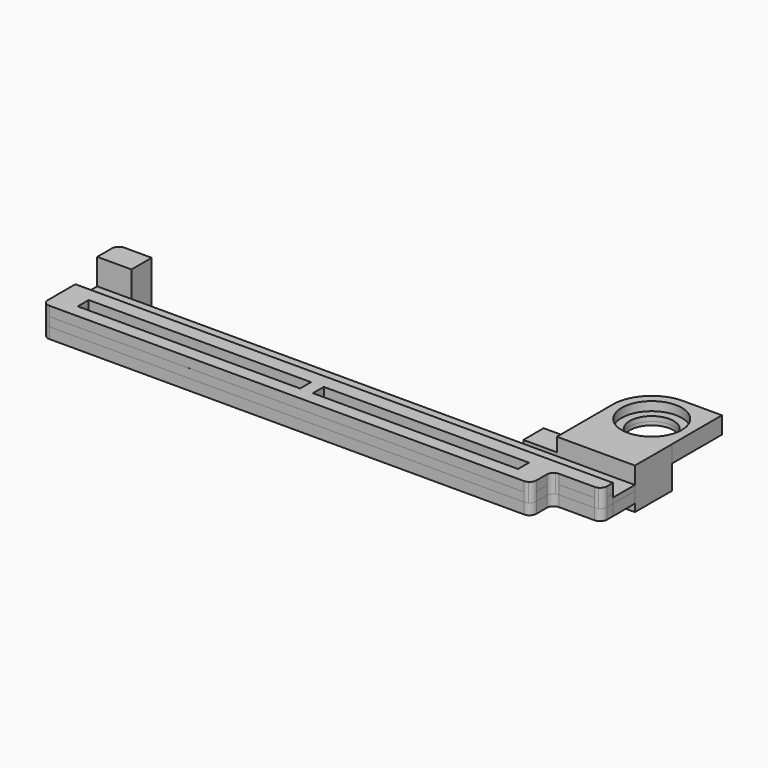
from build123d import *

# Parameters (mm, degrees)
F0_W           = 32.5
F0_H           = 2
F0_W_2         = 30
F1_DEPTH       = 1.4
F3_DEPTH       = 1.3
F4_DEPTH       = 1.6
F5_W           = 67
F5_H           = 6.7
F6_DEPTH       = 4.301
F9_T4_DEPTH    = 3.9
F9_T9_DEPTH    = 3.8
F9_T11_DEPTH   = 6.3
F9_T13_DEPTH   = 6.4
F9_2_F1_R      = 1
F9_2_F2_R      = 1
F11_DEPTH      = 4
F12_R          = 4.4
F13_DEPTH      = 2
F12_R_2        = 3.2
F14_DEPTH      = 0.7
F15_DEPTH      = 0.5
F7_W           = 5
F7_H           = 3.7
F16_DEPTH      = 3.3
F16_DEPTH_BACK = 2.9
F8_W           = 4.9
F8_H           = 3.7
F17_DEPTH      = 6
F19_DEPTH      = 0.5
F20_R          = 1


# Not quite as in the source:
# - a fillet or chamfer that OpenCascade refuses, or shapes differently, is made with other operations: its cross-section is extruded or revolved along the edge and cut away or added
# - ends of sketch curves that miss each other by under 0.0002 mm in the source are joined


with BuildPart() as f1:
    # F0 (on Top) → F1 (new body)
    with BuildSketch(Plane.XY):
        Polygon((78.6000193149, 6.0000242492), (1.93149e-05, 6.0000242492), (1.93149e-05, 2.42492e-05), (71.4000193149, 2.42492e-05), (71.4000193149, 3.9000242492), (78.6000193149, 3.9000242492), align=None)
        with Locations((19.8820251949, 2.9000242492)):
            Rectangle(F0_W, F0_H, mode=Mode.SUBTRACT)
        with Locations((52.9996412504, 2.9000242492)):
            Rectangle(F0_W_2, F0_H, mode=Mode.SUBTRACT)
    extrude(amount=F1_DEPTH)

    # F2 (on Top) → F3 (join)
    with BuildSketch(Plane.XY):
        with BuildLine():
            Line((-6.4456e-05, 6.0000242492), (-6.4456e-05, -2.57419e-05))
            Line((-6.4456e-05, -2.57419e-05), (71.399935544, -2.57419e-05))
            Line((71.399935544, -2.57419e-05), (71.399935544, 3.8999804767))
            Line((71.399935544, 3.8999804767), (78.599935544, 3.8999804767))
            Line((78.599935544, 3.8999804767), (78.599935544, 6.0000242492))
            add(Edge.make_bspline(
                [(78.599935544, 6.0000242492), (52.4000193149, 6.0000242492), (26.2000193149, 6.0000242492), (-6.4456e-05, 6.0000242492)],
                knots=[0, 0, 0, 0, 1, 1, 1, 1], degree=3))
        make_face()
        with BuildLine():
            Line((-6.4456e-05, 9.9999804767), (-6.4456e-05, 6.0000242492))
            add(Edge.make_bspline(
                [(78.6000193149, 6.0000242492), (52.4000193149, 6.0000242492), (26.2000193149, 6.0000242492), (-6.4456e-05, 6.0000242492)],
                knots=[0, 0, 0, 0, 1, 1, 1, 1], degree=3))
            Line((78.6000193149, 6.0000242492), (78.599935544, 9.9999804767))
            Line((78.599935544, 9.9999804767), (-6.4456e-05, 9.9999804767))
        make_face()
    extrude(amount=-F3_DEPTH)


with BuildPart() as f4:
    # F4 (new): a face of the model
    f4_faces = [f1.part.faces().sort_by_distance(p)[0] for p in [
        (37.9773022777, 5.1129767056, -1.3),
    ]]
    extrude(f4_faces, amount=F4_DEPTH)

    # F5 (on face) → F6 (cut, through all)
    with BuildSketch(Plane(origin=(0, 0, -2.9), x_dir=(1, 0, 0), z_dir=(0, 0, -1))):
        with Locations((35.6888609044, -4.8779113121)):
            Rectangle(F5_W, F5_H)
    extrude(amount=-F6_DEPTH, mode=Mode.SUBTRACT)

    # F9#2: fillet of radius 1 on 8 edges, made by hand

    # F9_2_f1
    f9_2_f1_edges = [f4.edges().sort_by_distance(p)[0] for p in [
        (71.399935544, 3.8999804767, -2.1),
        (69.1888609044, 8.2279113121, -2.1),
        (69.1888609044, 1.5279113121, -2.1),
        (2.1888609044, 8.2279113121, -2.1),
        (2.1888609044, 1.5279113121, -2.1),
    ]]
    fillet(f9_2_f1_edges, radius=F9_2_F1_R)

    # F9_2_f2
    f9_2_f2_edges = [f4.edges().sort_by_distance(p)[0] for p in [
        (71.399935544, -2.57419e-05, -2.1),
        (78.599935544, 3.8999804767, -2.1),
        (-6.4456e-05, -2.57419e-05, -2.1),
    ]]
    fillet(f9_2_f2_edges, radius=F9_2_F2_R)


with BuildPart() as f1_1:
    add(f1.part)

    # F9: fillet of radius 1 on 8 edges, made by hand


with BuildPart() as f9_tool2:
    # F9_s3 → F9_t4 (new body)
    with BuildSketch(Plane.XY.offset(-2.5)):
        with BuildLine():
            ThreePointArc((72.4000193149, 3.9000242492), (71.6929125337, 3.6071310304), (71.4000193149, 2.9000242492))
            Line((71.4000193149, 2.9000242492), (71.4000193149, 3.9000242492))
            Line((71.4000193149, 3.9000242492), (72.4000193149, 3.9000242492))
        make_face()
    extrude(amount=F9_T4_DEPTH)

    split(bisect_by=Plane.XY.offset(-1.3), keep=Keep.TOP)


with BuildPart() as f1_2:
    add(f1_1.part)

    # F9_t1: union F9_tool2
    add(f9_tool2.part)


with BuildPart() as f9_tool7:
    # F9_s8 → F9_t9 (new body)
    with BuildSketch(Plane.XY.offset(2.5)):
        with BuildLine():
            ThreePointArc((71.399935544, 2.8999804767), (71.6928287629, 3.6070872579), (72.399935544, 3.8999804767))
            Line((72.399935544, 3.8999804767), (71.399935544, 3.8999804767))
            Line((71.399935544, 3.8999804767), (71.399935544, 2.8999804767))
        make_face()
    extrude(amount=-F9_T9_DEPTH)

    split(bisect_by=Plane.XY.offset(1.4), keep=Keep.BOTTOM)


with BuildPart() as f1_3:
    add(f1_2.part)

    # F9_t6: union F9_tool7
    add(f9_tool7.part)

    # F9_s12 → F9_t11 (cut)
    with BuildSketch(Plane.XY.offset(-3.8)):
        with BuildLine():
            ThreePointArc((71.399935544, 0.9999742581), (71.1070423252, 0.292867477), (70.399935544, -2.57419e-05))
            Line((70.399935544, -2.57419e-05), (71.399935544, -2.57419e-05))
            Line((71.399935544, -2.57419e-05), (71.399935544, 0.9999742581))
        make_face()
        with BuildLine():
            ThreePointArc((78.599935544, 4.8999804767), (78.3070423252, 4.1928736955), (77.599935544, 3.8999804767))
            Line((77.599935544, 3.8999804767), (78.599935544, 3.8999804767))
            Line((78.599935544, 3.8999804767), (78.599935544, 4.8999804767))
        make_face()
        with BuildLine():
            ThreePointArc((-6.4456e-05, 0.9999742581), (0.2928287629, 0.292867477), (0.999935544, -2.57419e-05))
            Line((0.999935544, -2.57419e-05), (-6.4456e-05, -2.57419e-05))
            Line((-6.4456e-05, -2.57419e-05), (-6.4456e-05, 0.9999742581))
        make_face()
    extrude(amount=F9_T11_DEPTH, mode=Mode.SUBTRACT)

    # F9_s14 → F9_t13 (cut)
    with BuildSketch(Plane.XY.offset(-2.5)):
        with BuildLine():
            ThreePointArc((70.4000193149, 2.42492e-05), (71.1071260961, 0.292917468), (71.4000193149, 1.0000242492))
            Line((71.4000193149, 1.0000242492), (71.4000193149, 2.42492e-05))
            Line((71.4000193149, 2.42492e-05), (70.4000193149, 2.42492e-05))
        make_face()
        with BuildLine():
            ThreePointArc((78.6000193149, 4.9000242492), (78.3071260961, 4.192917468), (77.6000193149, 3.9000242492))
            Line((77.6000193149, 3.9000242492), (78.6000193149, 3.9000242492))
            Line((78.6000193149, 3.9000242492), (78.6000193149, 4.9000242492))
        make_face()
        with BuildLine():
            ThreePointArc((1.93149e-05, 1.0000242492), (0.2929125337, 0.292917468), (1.0000193149, 2.42492e-05))
            Line((1.0000193149, 2.42492e-05), (1.93149e-05, 2.42492e-05))
            Line((1.93149e-05, 2.42492e-05), (1.93149e-05, 1.0000242492))
        make_face()
    extrude(amount=F9_T13_DEPTH, mode=Mode.SUBTRACT)

    # F18 (on face) → F19 (cut)
    with BuildSketch(Plane.XY):
        with BuildLine():
            Line((78.599935544, 9.9999804767), (-6.4456e-05, 9.9999804767))
            Line((-6.4456e-05, 9.9999804767), (-6.4456e-05, 6.0000242492))
            add(Edge.make_bspline(
                [(-6.4456e-05, 6.0000242492), (26.2000193149, 6.0000242492), (52.4000193149, 6.0000242492), (78.6000193149, 6.0000242492)],
                knots=[0, 0, 0, 0, 1, 1, 1, 1], degree=3))
            Line((78.6000193149, 6.0000242492), (78.599935544, 9.9999804767))
        make_face()
    extrude(amount=-F19_DEPTH, mode=Mode.SUBTRACT)


with BuildPart() as f11:
    # F10 (on Top) → F11 (new body)
    with BuildSketch(Plane.XY):
        with BuildLine():
            Line((78.599935544, 9.9999804767), (78.6198350713, 16.7795400161))
            ThreePointArc((78.6198350713, 16.7795400161), (76.299661596, 14.5297660466), (73.1743396044, 13.7069353726))
            Line((73.1743396044, 13.7069353726), (67.1999678016, 13.7000184029))
            Line((67.1999678016, 13.7000184029), (67.1999678016, 10.0000184029))
            Line((67.1999678016, 10.0000184029), (78.599935544, 9.9999804767))
        make_face()
    extrude(amount=-F11_DEPTH)

    # F12 (on Top) + F10 (on Top) → F13 (join)
    with BuildSketch(Plane.XY):
        with BuildLine():
            Line((78.5999745131, 25.9072966889), (72.8999745131, 25.9072966889))
            ThreePointArc((72.8999745131, 25.9072966889), (68.8694658603, 24.2378053416), (67.1999745131, 20.2072966889))
            Line((67.1999745131, 20.2072966889), (67.1999745131, 13.7000184029))
            Line((67.1999745131, 13.7000184029), (73.1743396044, 13.7069353726))
            ThreePointArc((73.1743396044, 13.7069353726), (76.2830339187, 14.5204167001), (78.5999745131, 16.7469652605))
            Line((78.5999745131, 16.7469652605), (78.5999745131, 25.9072966889))
        make_face()
        with Locations((72.8999819636, 20.2072966889)):
            Circle(F12_R, mode=Mode.SUBTRACT)
    with BuildSketch(Plane.XY):
        with BuildLine():
            Line((78.599935544, 9.9999804767), (78.6198350713, 16.7795400161))
            ThreePointArc((78.6198350713, 16.7795400161), (76.299661596, 14.5297660466), (73.1743396044, 13.7069353726))
            Line((73.1743396044, 13.7069353726), (67.1999678016, 13.7000184029))
            Line((67.1999678016, 13.7000184029), (67.1999678016, 10.0000184029))
            Line((67.1999678016, 10.0000184029), (78.599935544, 9.9999804767))
        make_face()
    extrude(amount=F13_DEPTH)

    # F12 (on Top) → F14 (join)
    with BuildSketch(Plane.XY):
        with Locations((72.8999819636, 20.2072966889)):
            Circle(F12_R)
        with Locations((72.8999819636, 20.2072966889)):
            Circle(F12_R_2, mode=Mode.SUBTRACT)
    extrude(amount=F14_DEPTH)

    # F12 (on Top) → F15 (join)
    with BuildSketch(Plane.XY):
        with BuildLine():
            Line((78.5999745131, 25.9072966889), (72.8999745131, 25.9072966889))
            ThreePointArc((72.8999745131, 25.9072966889), (68.8694658603, 24.2378053416), (67.1999745131, 20.2072966889))
            Line((67.1999745131, 20.2072966889), (67.1999745131, 13.7000184029))
            Line((67.1999745131, 13.7000184029), (73.1743396044, 13.7069353726))
            ThreePointArc((73.1743396044, 13.7069353726), (76.2830339187, 14.5204167001), (78.5999745131, 16.7469652605))
            Line((78.5999745131, 16.7469652605), (78.5999745131, 25.9072966889))
        make_face()
        with Locations((72.8999819636, 20.2072966889)):
            Circle(F12_R, mode=Mode.SUBTRACT)
        with Locations((72.8999819636, 20.2072966889)):
            Circle(F12_R)
        with Locations((72.8999819636, 20.2072966889)):
            Circle(F12_R_2, mode=Mode.SUBTRACT)
    extrude(amount=-F15_DEPTH)


with BuildPart() as f16:
    # F7 (on Top) → F16 (new body, two sides)
    with BuildSketch(Plane.XY) as f16_sk:
        with Locations((2.5, 11.8499671802)):
            Rectangle(F7_W, F7_H)
    extrude(amount=F16_DEPTH)
    extrude(f16_sk.sketch, amount=-F16_DEPTH_BACK)

    # F20
    f20_edges = [f16.edges().sort_by_distance(p)[0] for p in [
        (0, 13.699967, 0.2),
    ]]
    fillet(f20_edges, radius=F20_R)


with BuildPart() as f17:
    # F8 (on face) → F17 (new body)
    with BuildSketch(Plane.XY):
        with Locations((64.7499678016, 11.8500184029)):
            Rectangle(F8_W, F8_H)
    extrude(amount=-F17_DEPTH)


solid = Compound([f4.part, f1_3.part, f11.part, f16.part, f17.part])
